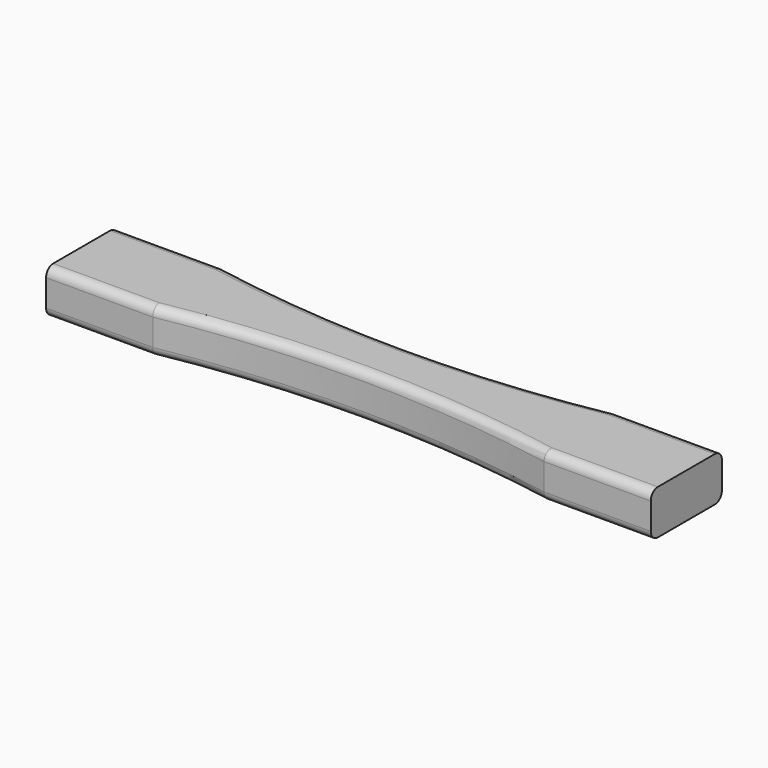
from build123d import *

# Parameters (mm, degrees)
F0_W     = 60
F0_H     = 50
F0_W_2   = 60.0000097896
F1_DEPTH = 25
F2_R     = 5


# Not quite as in the source:
# - ends of sketch curves that miss each other by under 0.0002 mm in the source are joined


with BuildPart() as f1:
    # F0 (on Top) → F1 (new body)
    with BuildSketch(Plane.XY):
        with Locations((-140, 0)):
            Rectangle(F0_W, F0_H)
        with BuildLine():
            Line((-110, 25), (-110, -25))
            ThreePointArc((-110, -25), (-4.8948e-06, -15), (109.9999902104, -25))
            Line((109.9999902104, -25), (109.9999902104, 25))
            ThreePointArc((109.9999902104, 25), (0, 14.9999991026), (-110, 25))
        make_face()
        with Locations((139.9999951052, 0)):
            Rectangle(F0_W_2, F0_H)
    extrude(amount=F1_DEPTH)

    # F2
    f2_edges = [f1.edges().sort_by_distance(p)[0] for p in [
        (-140, -25, 25),
        (-5e-06, -15, 25),
        (139.999995, -25, 25),
        (139.999995, 25, 25),
        (-5e-06, 14.999999, 25),
        (-140, 25, 25),
        (-140, -25, 0),
        (-5e-06, -15, 0),
        (139.999995, -25, 0),
        (-140, 25, 0),
        (-5e-06, 14.999999, 0),
        (139.999995, 25, 0),
    ]]
    fillet(f2_edges, radius=F2_R)


solid = f1.part
